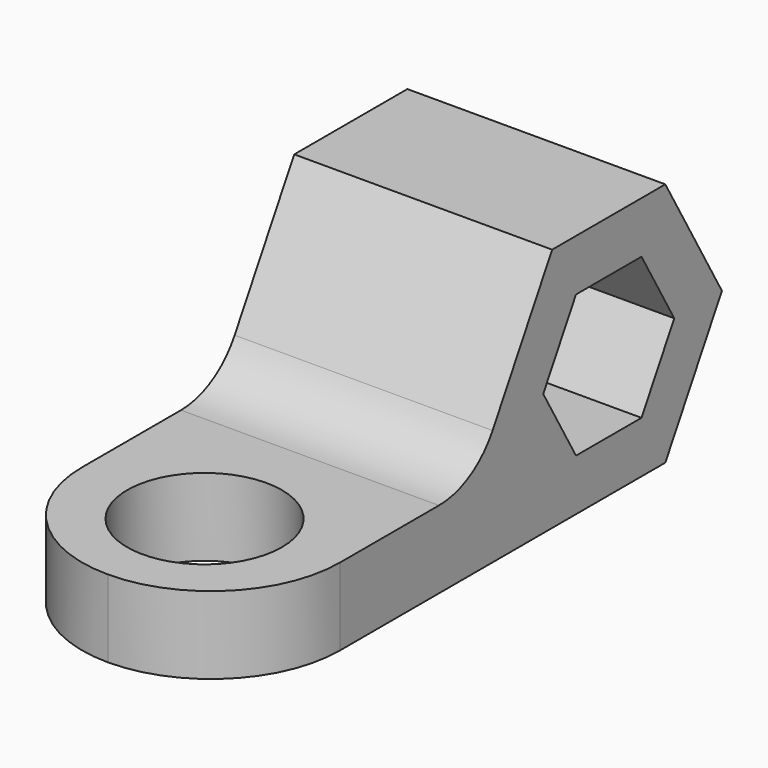
from build123d import *

# Parameters (mm, degrees)
F1_DEPTH    = 10
F2_R        = 3
F3_DEPTH    = 25
F4_R        = 4.99999
F5_T1_DEPTH = 10


# Not quite as in the source:
# - a fillet or chamfer that OpenCascade refuses, or shapes differently, is made with other operations: its cross-section is extruded or revolved along the edge and cut away or added
# - a fillet or chamfer is up to 0.001 mm smaller than in the source, because OpenCascade refuses the exact size


with BuildPart() as f1:
    # F0 (on Right) → F1 (new body)
    with BuildSketch(Plane.YZ):
        Polygon((-20.7655076647, 0), (0, 0), (2.7424137787, 4.75), (0, 9.5), (-5.4848275573, 9.5), (-8.3715789032, 4.5), (-8.3715789032, 3), (-20.7655076647, 3), align=None)
        Polygon((-4.3301270189, 2), (-5.9178402592, 4.75), (-4.3301270189, 7.5), (-1.1547005384, 7.5), (0.4330127019, 4.75), (-1.1547005384, 2), align=None, mode=Mode.SUBTRACT)
    extrude(amount=F1_DEPTH)

    # F2 (on face) → F3 (cut)
    with BuildSketch(Plane.XY.offset(3)):
        with Locations((5, -16.0806495696)):
            Circle(F2_R)
    extrude(amount=-F3_DEPTH, mode=Mode.SUBTRACT)

    # F4 (radius 5 in the source; OpenCascade refuses exactly that, so slightly less here)
    f4_edges = [f1.edges().sort_by_distance(p)[0] for p in [
        (0, -20.765508, 1.5),
        (10, -20.765508, 1.5),
    ]]
    fillet(f4_edges, radius=F4_R)

    # F5: fillet of radius 3 on 1 edges, made by hand

    # F5_s2 → F5_t1 (join)
    with BuildSketch(Plane.YZ):
        with BuildLine():
            ThreePointArc((-10.9696551146, 3), (-9.4696551146, 3.4019237886), (-8.3715789032, 4.5))
            Line((-8.3715789032, 4.5), (-8.3715789032, 3))
            Line((-8.3715789032, 3), (-10.9696551146, 3))
        make_face()
    extrude(amount=F5_T1_DEPTH)


solid = f1.part
